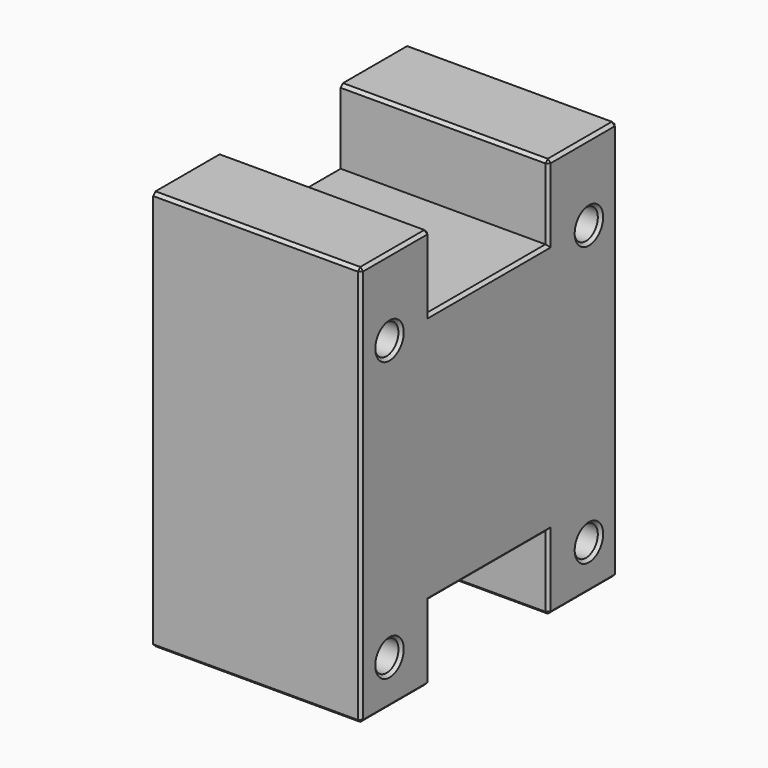
from build123d import *

# Parameters (mm, degrees)
F1_DEPTH = 70
F2_R     = 8
F3_DEPTH = 10
F4_R     = 5
F5_DEPTH = 70.001
F6_SIZE  = 1


# Not quite as in the source:
# - a feature names something its author has since deleted; it is built from what else it names


with BuildPart() as f1:
    # F0 (on Right) → F1 (new body)
    with BuildSketch(Plane.YZ):
        Polygon((-25, 67.5), (-54, 67.5), (-54, -67.5), (-25, -67.5), (-25, -42.5), (25, -42.5), (25, -67.5), (54, -67.5), (54, 67.5), (25, 67.5), (25, 42.5), (-25, 42.5), align=None)
    extrude(amount=F1_DEPTH)

    # F2 (on face) → F3 (cut)
    with BuildSketch(Plane(origin=(0, 0, 0), x_dir=(0, -1, 0), z_dir=(-1, 0, 0))):
        with Locations((41.9203005731, 41.5)):
            Circle(F2_R)
        with Locations((-42.0796994269, 41.5)):
            Circle(F2_R)
        with Locations((41.9203005731, -52.5)):
            Circle(F2_R)
        with Locations((-42.0796994269, -52.5)):
            Circle(F2_R)
    extrude(amount=-F3_DEPTH, mode=Mode.SUBTRACT)

    # F4 (on face) → F5 (cut, through all)
    with BuildSketch(Plane(origin=(0, 0, 0), x_dir=(0, -1, 0), z_dir=(-1, 0, 0))):
        with Locations((-42.0796994269, 41.5)):
            Circle(F4_R)
        with Locations((41.9203005731, 41.5)):
            Circle(F4_R)
        with Locations((41.9203005731, -52.5)):
            Circle(F4_R)
        with Locations((-42.0796994269, -52.5)):
            Circle(F4_R)
    extrude(amount=-F5_DEPTH, mode=Mode.SUBTRACT)

    # F6
    f6_edges = [f1.edges().sort_by_distance(p)[0] for p in [
        (70, -39.5, 67.5),
        (70, -25, 55),
        (70, -54, 0),
        (70, 0, 42.5),
        (70, -39.5, -67.5),
        (70, 25, 55),
        (70, -25, -55),
        (70, 39.5, 67.5),
        (70, 0, -42.5),
        (70, 54, 0),
        (70, 25, -55),
        (70, 39.5, -67.5),
        (70, -36.920301, -52.5),
        (70, 47.079699, -52.5),
        (70, -36.920301, 41.5),
        (70, 47.079699, 41.5),
        (35, -54, -67.5),
        (35, -25, -67.5),
        (35, 25, -67.5),
        (35, 54, -67.5),
        (35, -54, 67.5),
        (35, -25, 67.5),
        (35, 25, 67.5),
        (35, 54, 67.5),
    ]]
    chamfer(f6_edges, length=F6_SIZE)


solid = f1.part
